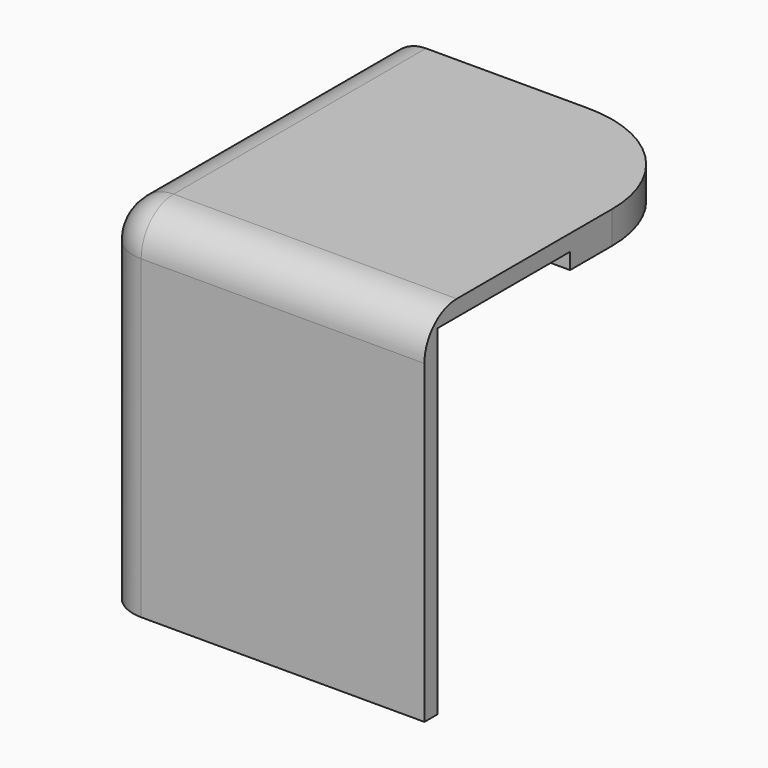
from build123d import *

# Parameters (mm, degrees)
F0_W      = 40
F0_H      = 44
F1_DEPTH  = 44
F2_W      = 40
F2_H      = 40
F3_DEPTH  = 36
F5_DEPTH  = 5
F7_DEPTH  = 5
F8_R      = 15
F9_R      = 5
F11_DEPTH = 5


# Not quite as in the source:
# - a feature names something its author has since deleted; it is built from what else it names


with BuildPart() as f1:
    # F0 (on Top) → F1 (new body)
    with BuildSketch(Plane.XY):
        with Locations((20, 22)):
            Rectangle(F0_W, F0_H)
    extrude(amount=F1_DEPTH)

    # F2 (on face) → F3 (cut)
    with BuildSketch(Plane.YZ.offset(40)):
        with Locations((24, 20)):
            Rectangle(F2_W, F2_H)
    extrude(amount=-F3_DEPTH, mode=Mode.SUBTRACT)

    # F4 (on face) → F5 (cut)
    with BuildSketch(Plane.YZ.offset(40)):
        Polygon((2, 42), (2, 0), (4, 0), (4, 40), (22.5, 40), (22.5, 42), align=None)
    extrude(amount=-F5_DEPTH, mode=Mode.SUBTRACT)

    # F6 (on face) → F7 (cut)
    with BuildSketch(Plane(origin=(0, 44, 0), x_dir=(-1, 0, 0), z_dir=(0, 1, 0))):
        Polygon((-4, 40), (-4, 0), (-2, 0), (-2, 42), (-22.5, 42), (-22.5, 40), align=None)
    extrude(amount=-F7_DEPTH, mode=Mode.SUBTRACT)

    # F8
    f8_edges = [f1.edges().sort_by_distance(p)[0] for p in [
        (40, 44, 42),
    ]]
    fillet(f8_edges, radius=F8_R)

    # F9
    f9_edges = [f1.edges().sort_by_distance(p)[0] for p in [
        (0, 22, 44),
        (20, 0, 44),
        (0, 0, 22),
    ]]
    fillet(f9_edges, radius=F9_R)

    # F10 (on face) → F11 (cut)
    with BuildSketch(Plane(origin=(0, 0, 0), x_dir=(1, 0, 0), z_dir=(0, 0, -1))):
        Polygon((35, -4), (35, -2), (2, -2), (2, -39), (4, -39), (4, -4), align=None)
    extrude(amount=-F11_DEPTH, mode=Mode.SUBTRACT)


solid = f1.part
